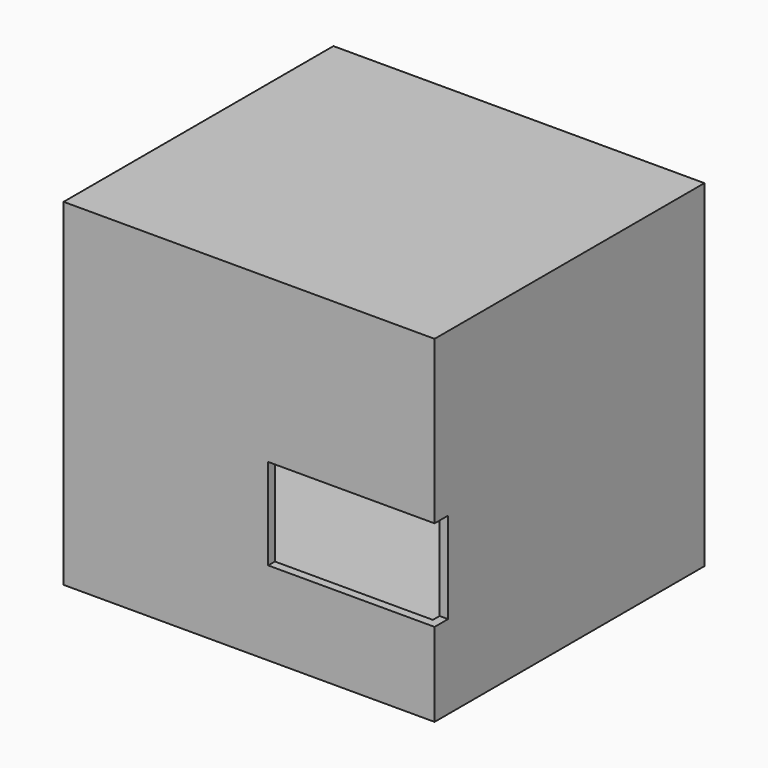
from build123d import *

# Parameters (mm, degrees)
F0_W     = 558.8
F0_H     = 508
F1_DEPTH = 508
F2_T     = -12.7
F5_W     = 250.6727086544
F5_H     = 137.283227253
F6_DEPTH = 25.4


# Not quite as in the source:
# - the program builds the solid bodies; features that only make, move or delete a surface that nothing else refers to are left out


with BuildPart() as f1:
    # F0 (on Front) → F1 (new body)
    with BuildSketch(Plane.XZ):
        with Locations((-279.4, -328.6047284609)):
            Rectangle(F0_W, F0_H)
    extrude(amount=F1_DEPTH)

    # F2
    f2_openings = [f1.faces().sort_by_distance(p)[0] for p in [
        (-558.8, -254, -328.604728),
    ]]
    offset(amount=F2_T, openings=f2_openings)

    # F5 (on face) → F6 (cut)
    with BuildSketch(Plane.XZ.offset(508)):
        with Locations((-125.3363543272, -387.9528045654)):
            Rectangle(F5_W, F5_H)
    extrude(amount=-F6_DEPTH, mode=Mode.SUBTRACT)


solid = f1.part
